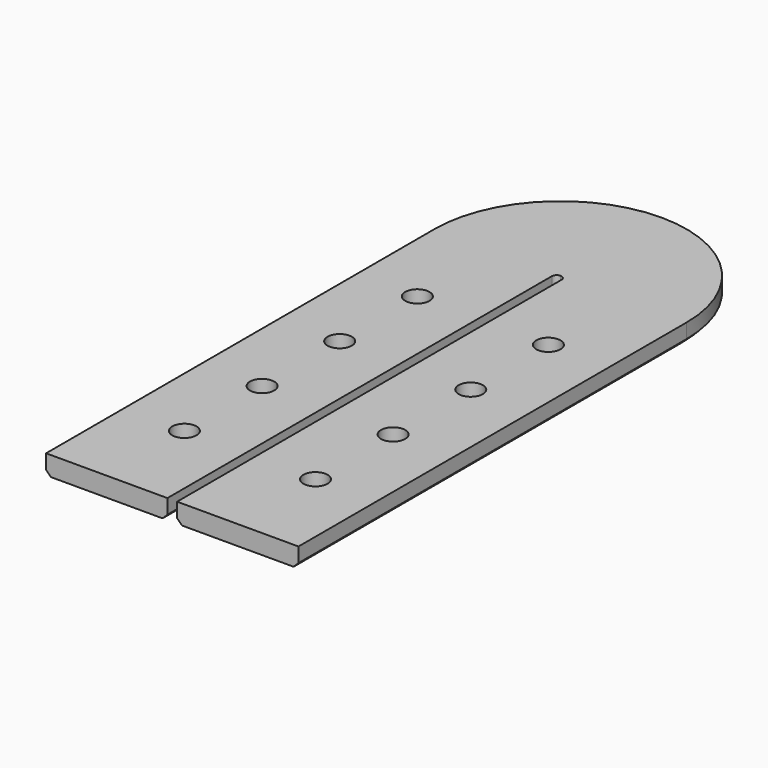
from build123d import *

# Parameters (mm, degrees)
F0_R     = 125
F1_DEPTH = 200
F2_SIZE  = 50
F3_R     = 49.99999


# Not quite as in the source:
# - a fillet or chamfer is up to 0.001 mm smaller than in the source, because OpenCascade refuses the exact size


with BuildPart() as f1:
    # F0 (on Top) → F1 (new body)
    with BuildSketch(Plane.XY):
        with BuildLine():
            Line((-50, 0), (0, 0))
            Line((0, 0), (50, 0))
            Line((50, 0), (50, -5000))
            Line((50, -5000), (1300, -5000))
            Line((1300, -5000), (1300, 0))
            ThreePointArc((1300, 0), (0, 1300), (-1300, 0))
            Line((-1300, 0), (-1300, -5000))
            Line((-1300, -5000), (-50, -5000))
            Line((-50, -5000), (-50, 0))
        make_face()
        with Locations((-675, -4000)):
            Circle(F0_R, mode=Mode.SUBTRACT)
        with Locations((-675, -3000)):
            Circle(F0_R, mode=Mode.SUBTRACT)
        with Locations((-675, -2000)):
            Circle(F0_R, mode=Mode.SUBTRACT)
        with Locations((675, -4000)):
            Circle(F0_R, mode=Mode.SUBTRACT)
        with Locations((675, -3000)):
            Circle(F0_R, mode=Mode.SUBTRACT)
        with Locations((675, -2000)):
            Circle(F0_R, mode=Mode.SUBTRACT)
        with Locations((-675, -1000)):
            Circle(F0_R, mode=Mode.SUBTRACT)
        with Locations((675, -1000)):
            Circle(F0_R, mode=Mode.SUBTRACT)
    extrude(amount=F1_DEPTH)

    # F2
    f2_edges = [f1.edges().sort_by_distance(p)[0] for p in [
        (1300, -2500, 0),
        (0, 1300, 0),
        (-1300, -2500, 0),
        (50, -2500, 0),
        (-50, -2500, 0),
        (0, 0, 0),
    ]]
    chamfer(f2_edges, length=F2_SIZE)

    # F3 (radius 50 in the source; OpenCascade refuses exactly that, so slightly less here)
    f3_edges = [f1.edges().sort_by_distance(p)[0] for p in [
        (-50, 0, 125),
        (50, 0, 125),
    ]]
    fillet(f3_edges, radius=F3_R)


solid = f1.part
